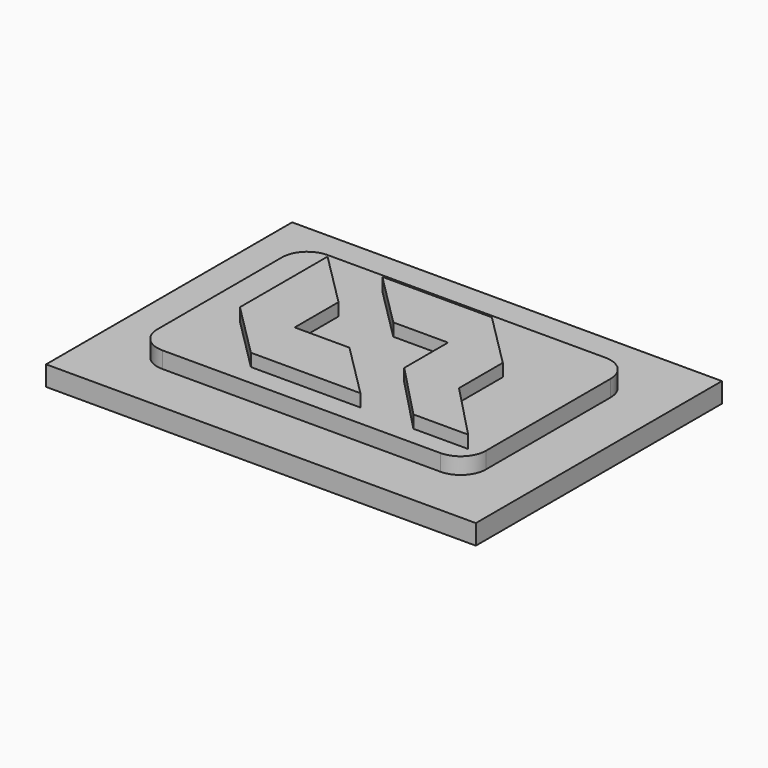
from build123d import *

# Parameters (mm, degrees)
F3_DEPTH = 1.651
F4_DEPTH = 1.27
F5_W     = 43.18
F5_H     = 30.902041302
F6_DEPTH = 2


with BuildPart() as f3:
    # F2 (on face) → F3 (new body)
    with BuildSketch(Plane.XY):
        with BuildLine():
            Line((15.24, 32.0904812722), (-12.7, 32.0904812722))
            ThreePointArc((-12.7, 32.0904812722), (-14.4960512242, 31.3465324964), (-15.24, 29.5504812722))
            Line((-15.24, 29.5504812722), (-15.24, 13.8884399702))
            ThreePointArc((-15.24, 13.8884399702), (-14.4960512242, 12.092388746), (-12.7, 11.3484399702))
            Line((-12.7, 11.3484399702), (15.24, 11.3484399702))
            ThreePointArc((15.24, 11.3484399702), (17.0360512242, 12.092388746), (17.78, 13.8884399702))
            Line((17.78, 13.8884399702), (17.78, 29.5504812722))
            ThreePointArc((17.78, 29.5504812722), (17.0360512242, 31.3465324964), (15.24, 32.0904812722))
        make_face()
    extrude(amount=-F3_DEPTH)

    # F1 (on face) → F4 (join)
    with BuildSketch(Plane.XY):
        Polygon((-5.502041302, 24.4704812722), (-11.0040826039, 29.9725225741), (-11.0040826039, 18.9684399702), (-5.502041302, 13.4663986682), (5.502041302, 13.4663986682), (0, 18.9684399702), (-5.502041302, 18.9684399702), align=None)
        Polygon((5.502041302, 29.9725225741), (-5.502041302, 29.9725225741), (0, 24.4704812722), (5.502041302, 24.4704812722), (5.502041302, 18.9684399702), (11.0040826039, 13.245652739), (16.5061239059, 13.245652739), (11.0040826039, 18.9684399702), (11.0040826039, 24.4704812722), align=None)
    extrude(amount=F4_DEPTH)

    # F5 (on face) → F6 (join)
    with BuildSketch(Plane(origin=(0, 0, -1.651), x_dir=(1, 0, 0), z_dir=(0, 0, -1))):
        with Locations((1.27, -21.7194606212)):
            Rectangle(F5_W, F5_H)
    extrude(amount=F6_DEPTH)


solid = f3.part
